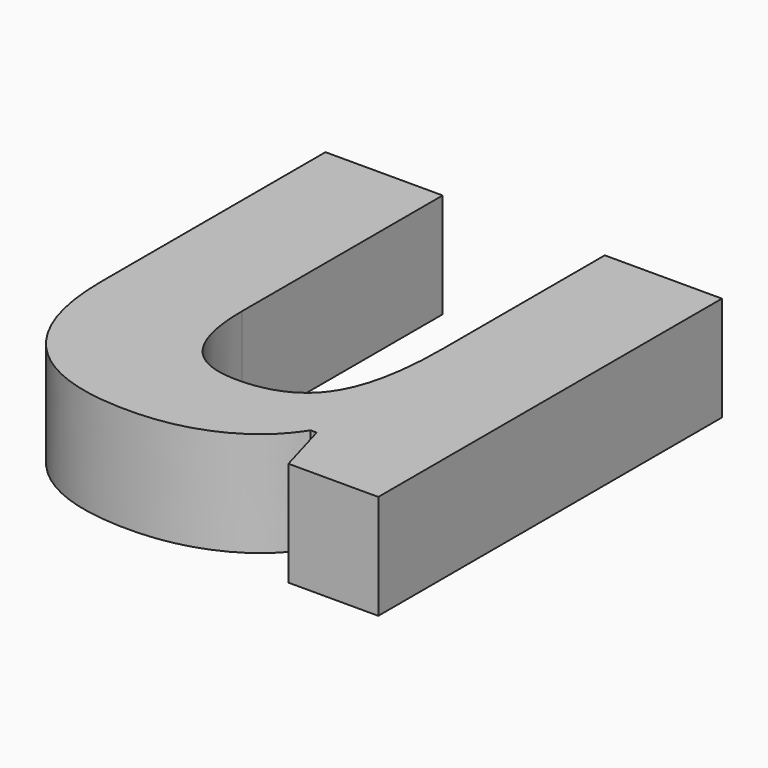
from build123d import *

# Parameters (mm, degrees)
F0_TEXT_SIZE = 75.1475079192
F1_DEPTH     = 10


# Not quite as in the source:
# - Text() gives the source's letters only with a copy of the font that has no kerning and outlines rounded to 1/6400 em; it was checked with that copy


with BuildPart() as f1:
    # F0 (on Top) → F1 (new body)
    with BuildSketch(Plane.XY):
        with Locations((0, 0)):
            Text('u', F0_TEXT_SIZE, font='Open Sans', font_style=FontStyle.BOLD, text_align=(TextAlign.LEFT, TextAlign.BOTTOM))
    extrude(amount=F1_DEPTH)


solid = f1.part
